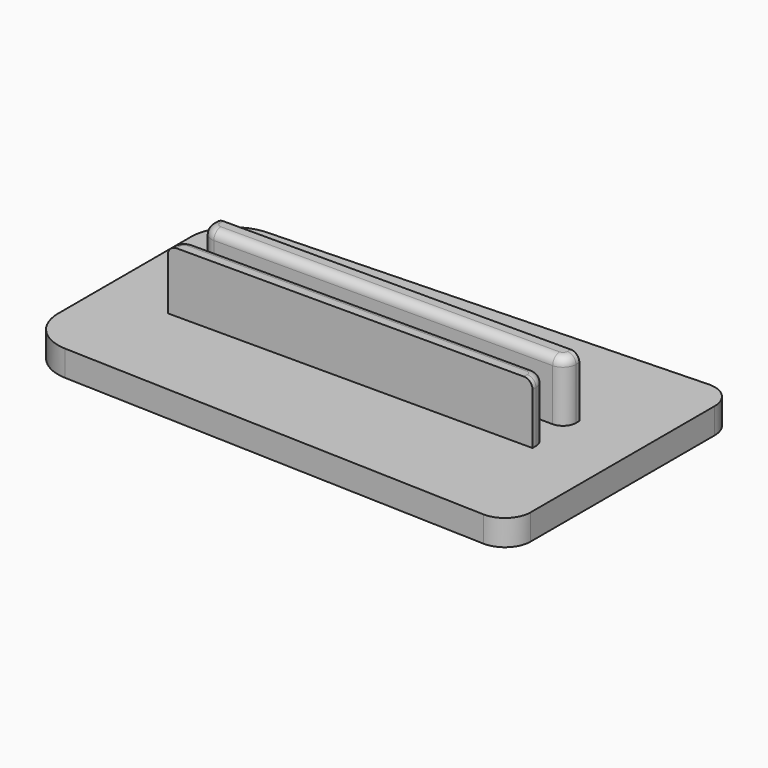
from build123d import *

# Parameters (mm, degrees)
F0_W     = 42.4481438452
F0_H     = 2
F1_DEPTH = 3
F2_DEPTH = 10
F3_R     = 1.5
F4_R     = 1
F5_R     = 3
F6_R     = 5


with BuildPart() as f1:
    # F0 (on Top) → F1 (new body)
    with BuildSketch(Plane.XY):
        Polygon((-65.7136544558, 49.5634722376), (-65.7136544558, 36.4734722376), (-65.7136544558, 35.0634722376), (-65.7136544558, 33.6534722376), (-65.7136544558, 20.5634722376), (-7.7136544558, 18.5634722376), (-7.7136544558, 51.5634722376), align=None)
        with Locations((-36.7136544558, 32.6534722376)):
            Rectangle(F0_W, F0_H, mode=Mode.SUBTRACT)
        with Locations((-36.7136544558, 37.4734722376)):
            Rectangle(F0_W, F0_H, mode=Mode.SUBTRACT)
    extrude(amount=F1_DEPTH)

    # F0 (on Top) → F2 (join)
    with BuildSketch(Plane.XY):
        with Locations((-36.7136544558, 32.6534722376)):
            Rectangle(F0_W, F0_H)
        with Locations((-36.7136544558, 37.4734722376)):
            Rectangle(F0_W, F0_H)
    extrude(amount=F2_DEPTH)

    # F3
    f3_edges = [f1.edges().sort_by_distance(p)[0] for p in [
        (-57.937726, 36.473472, 6.5),
        (-57.937726, 33.653472, 6.5),
        (-15.489583, 36.473472, 6.5),
        (-15.489583, 33.653472, 6.5),
    ]]
    fillet(f3_edges, radius=F3_R)

    # F4
    f4_edges = [f1.edges().sort_by_distance(p)[0] for p in [
        (-36.713654, 36.473472, 10),
        (-36.713654, 33.653472, 10),
        (-57.498387, 33.214132, 10),
        (-15.928922, 33.214132, 10),
        (-57.937726, 31.903472, 10),
        (-15.489583, 31.903472, 10),
        (-57.937726, 38.223472, 10),
        (-57.498387, 36.912812, 10),
        (-15.489583, 38.223472, 10),
        (-15.928922, 36.912812, 10),
    ]]
    fillet(f4_edges, radius=F4_R)

    # F5
    f5_edges = [f1.edges().sort_by_distance(p)[0] for p in [
        (-7.713654, 18.563472, 1.5),
        (-7.713654, 51.563472, 1.5),
    ]]
    fillet(f5_edges, radius=F5_R)

    # F6
    f6_edges = [f1.edges().sort_by_distance(p)[0] for p in [
        (-65.713654, 20.563472, 1.5),
        (-65.713654, 49.563472, 1.5),
    ]]
    fillet(f6_edges, radius=F6_R)


solid = f1.part
